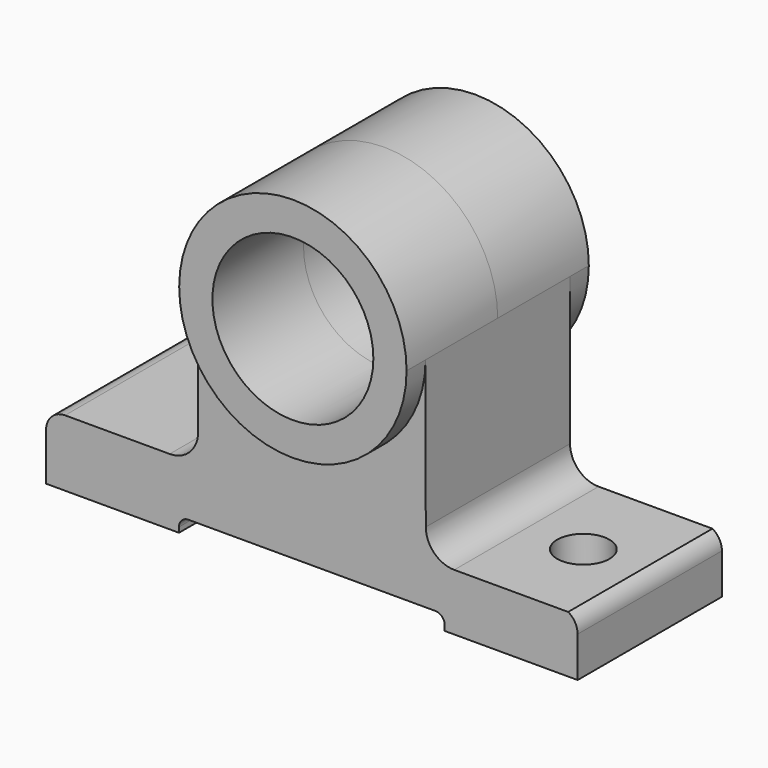
from build123d import *
from build123d import SkipClean  # not in build123d's __all__

# Parameters (mm, degrees)
F1_DEPTH = 30.1625
F0_R     = 26.9169820067
F2_DEPTH = 38.1
F6_D     = 4.7625
F6_DEPTH = 114.301
F7_D     = 17.4625
F7_DEPTH = 19.0282397391


with BuildPart() as f1:
    # F0 (on Front) → F1 (new body, symmetric)
    with BuildSketch(Plane.XZ):
        with BuildLine():
            ThreePointArc((41.2750103626, 4.8735072878), (43.5200676937, 3.9435676542), (44.4499999995, 1.6985072878))
            Line((44.4499999995, 1.6985072878), (44.4499999995, 0))
            Line((44.4499999995, 0), (88.8999999995, 0))
            Line((88.8999999995, 0), (88.8999999995, 13.5279764081))
            ThreePointArc((88.8999999995, 13.5279764081), (88.0492603051, 16.7029781548), (85.7249965061, 19.0272397391))
            Line((85.7249965061, 19.0272397391), (47.6269838993, 19.0272397391))
            ThreePointArc((47.6269838993, 19.0272397391), (40.8967892902, 21.812053872), (38.1019943796, 28.5381099704))
            Line((38.1019943796, 28.5381099704), (38.0289897107, 77.7511383134))
            ThreePointArc((38.0289897107, 77.7511383134), (-2e-10, 39.7221486024), (-38.0289897112, 77.7511383134))
            Line((-38.0289897112, 77.7511383134), (-38.0289897112, 31.7225298162))
            ThreePointArc((-38.0289897112, 31.7225298162), (-40.8187976204, 24.9873377254), (-47.5539897112, 22.1975298162))
            Line((-47.5539897112, 22.1975298162), (-82.55, 22.1975298162))
            ThreePointArc((-82.55, 22.1975298162), (-87.0401280605, 20.3376578767), (-88.9, 15.8475298162))
            Line((-88.9, 15.8475298162), (-88.9, 0))
            Line((-88.9, 0), (-44.45, 0))
            Line((-44.45, 0), (-44.45, 1.6987767268))
            ThreePointArc((-44.45, 1.6987767268), (-43.5200603664, 3.943844421), (-41.274989637, 4.8737767268))
            Line((-41.274989637, 4.8737767268), (41.2750103626, 4.8735072878))
        make_face()
    extrude(amount=F1_DEPTH, both=True)

    # F0 (on Front) → F2 (join, symmetric)
    with BuildSketch(Plane.XZ):
        with BuildLine():
            ThreePointArc((-38.0289897112, 77.7511383134), (-2e-10, 39.7221486024), (38.0289897107, 77.7511383134))
            ThreePointArc((38.0289897107, 77.7511383134), (-2e-10, 115.7801280244), (-38.0289897112, 77.7511383134))
        make_face()
        with Locations((-2e-10, 77.7511383134)):
            Circle(F0_R, mode=Mode.SUBTRACT)
    with SkipClean():  # cleaning this boolean's faces spoils the solid; the shape is the same uncleaned
        extrude(amount=F2_DEPTH, both=True)

    # F6 (through all, one way)
    with BuildSketch(Plane.XY.offset(114.3)):
        with Locations((0, 0)):
            Circle(F6_D / 2)
    extrude(amount=-F6_DEPTH, mode=Mode.SUBTRACT)

    # F7 (through all, one way)
    with BuildSketch(Plane.XY.offset(19.0272397391)):
        with Locations((-66.6769838993, 0), (66.6769838993, 0)):
            Circle(F7_D / 2)
    extrude(amount=-F7_DEPTH, mode=Mode.SUBTRACT)


solid = f1.part
